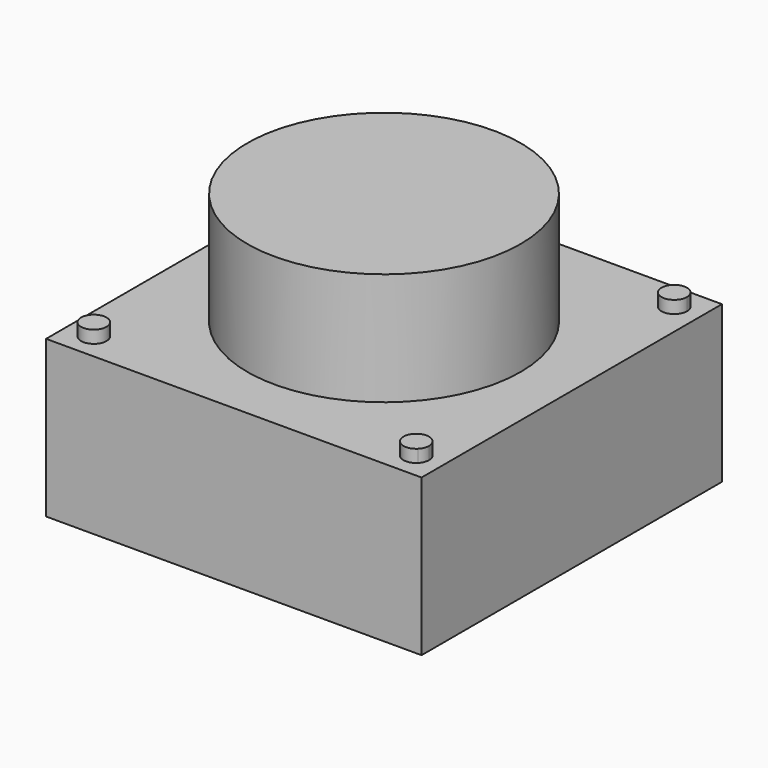
from build123d import *

# Parameters (mm, degrees)
F0_W     = 6
F0_H     = 6
F1_DEPTH = 2.5
F2_R     = 2.18397174
F3_DEPTH = 1.8
F2_R_2   = 0.2032
F4_DEPTH = 0.2


with BuildPart() as f1:
    # F0 (on Top) → F1 (new body)
    with BuildSketch(Plane.XY):
        with Locations((3, -3)):
            Rectangle(F0_W, F0_H)
    extrude(amount=F1_DEPTH)

    # F2 (on face) → F3 (join)
    with BuildSketch(Plane.XY.offset(2.5)):
        with Locations((3, -3)):
            Circle(F2_R)
    extrude(amount=F3_DEPTH)

    # F2 (on face) → F4 (join)
    with BuildSketch(Plane.XY.offset(2.5)):
        with BuildLine():
            ThreePointArc((0.6254458211, -0.4234319816), (0.5007393311, -0.23679553), (0.2805866258, -0.2805866258))
            ThreePointArc((0.2805866258, -0.2805866258), (0.2805866258, -0.5662773374), (0.5662773374, -0.5662773374))
            ThreePointArc((0.5662773374, -0.5662773374), (0.6100684332, -0.5007393311), (0.6254458211, -0.4234319816))
        make_face()
        with BuildLine():
            ThreePointArc((5.7797680184, -5.5765680184), (5.3888356974, -5.498806745), (5.7202521163, -5.7202521163))
            ThreePointArc((5.7202521163, -5.7202521163), (5.7643003394, -5.6543292919), (5.7797680184, -5.5765680184))
        make_face()
        with BuildLine():
            ThreePointArc((5.7797680184, -0.4234319816), (5.7643003394, -0.3456707081), (5.7202521163, -0.2797478837))
            ThreePointArc((5.7202521163, -0.2797478837), (5.3888356974, -0.501193255), (5.7797680184, -0.4234319816))
        make_face()
        with Locations((0.4234319816, -5.5765680184)):
            Circle(F2_R_2)
    extrude(amount=F4_DEPTH)


solid = f1.part
